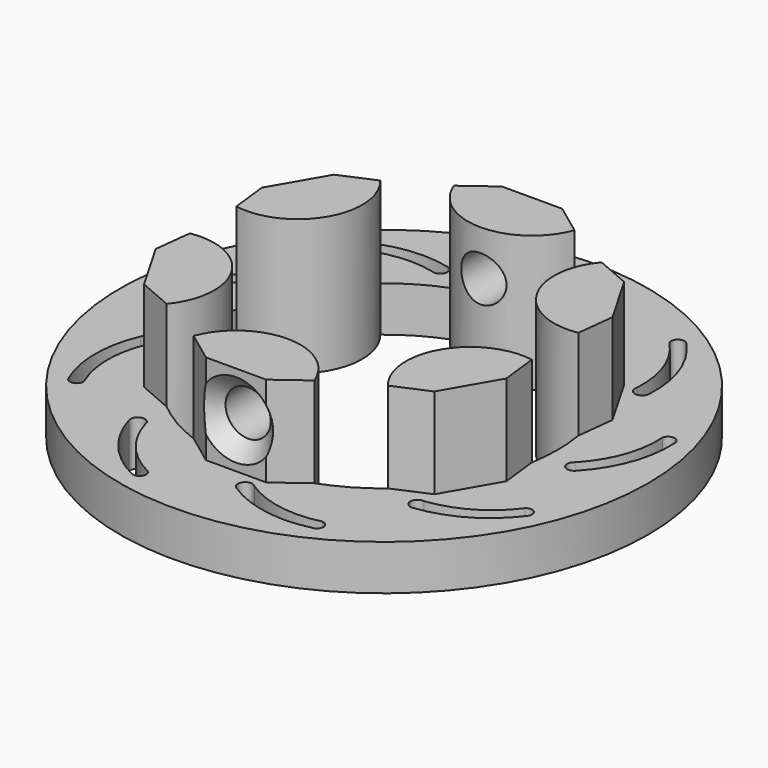
from build123d import *

# Parameters (mm, degrees)
F0_R          = 17.5
F0_R_2        = 11.5
F1_DEPTH      = 3
F3_DEPTH      = 3.001
F5_DEPTH      = 6
F5_DEPTH_BACK = 3
F6_R          = 1.5
F7_DEPTH      = 29.767666761


# Not quite as in the source:
# - a fillet or chamfer that OpenCascade refuses, or shapes differently, is made with other operations: its cross-section is extruded or revolved along the edge and cut away or added


with BuildPart() as f1:
    # F0 (on Top) → F1 (new body)
    with BuildSketch(Plane.XY):
        Circle(F0_R)
        Circle(F0_R_2, mode=Mode.SUBTRACT)
    extrude(amount=F1_DEPTH)

    # F2 (on Top) → F3 (cut, through all)
    with BuildSketch(Plane.XY):
        with BuildLine():
            ThreePointArc((10.3428791664, 8.0132342217), (10.722508829, 7.4074823165), (11.2842680034, 7.8496142891))
            ThreePointArc((11.2842680034, 7.8496142891), (10.8476709377, 10.9006538274), (9.2192751651, 13.5174813857))
            ThreePointArc((9.2192751651, 13.5174813857), (8.6315737781, 13.5584848298), (8.5342502168, 12.9774492654))
            ThreePointArc((8.5342502168, 12.9774492654), (9.9604845752, 10.6854945477), (10.3428791664, 8.0132342217))
        make_face()
        with BuildLine():
            ThreePointArc((2.7722974401, 12.7867681236), (3.4524804527, 12.5667564861), (3.5986159928, 13.2665410638))
            ThreePointArc((3.5986159928, 13.2665410638), (1.3029928249, 15.3231337636), (-1.6264950391, 16.2810273468))
            ThreePointArc((-1.6264950391, 16.2810273468), (-2.1030569267, 15.9346706376), (-1.8041286384, 15.427013193))
            ThreePointArc((-1.8041286384, 15.427013193), (0.761670361, 14.5880397916), (2.7722974401, 12.7867681236))
        make_face()
        with BuildLine():
            ThreePointArc((-6.0954730691, 11.5772311114), (-5.4330018975, 11.8459056319), (-5.770868435, 12.4759058335))
            ThreePointArc((-5.770868435, 12.4759058335), (-8.8513701119, 12.5757491141), (-11.711210138, 11.426499669))
            ThreePointArc((-11.711210138, 11.426499669), (-11.8536439226, 10.85484696), (-11.298335653, 10.6581061954))
            ThreePointArc((-11.298335653, 10.6581061954), (-8.7935378801, 11.6646790891), (-6.0954730691, 11.5772311114))
        make_face()
        with BuildLine():
            ThreePointArc((-12.1111039857, 4.9505789955), (-11.7763222787, 5.5822238799), (-12.440099386, 5.8476556095))
            ThreePointArc((-12.440099386, 5.8476556095), (-14.8640786012, 3.9440316902), (-16.3161198577, 1.2253858046))
            ThreePointArc((-16.3161198577, 1.2253858046), (-16.0577791885, 0.6959197515), (-15.5059258486, 0.9021528573))
            ThreePointArc((-15.5059258486, 0.9021528573), (-14.2341520178, 3.2832854023), (-12.1111039857, 4.9505789955))
        make_face()
        with BuildLine():
            ThreePointArc((-12.4598147474, -3.9925040519), (-12.6093705865, -3.293442465), (-13.288469578, -3.5167776637))
            ThreePointArc((-13.288469578, -3.5167776637), (-13.9217195173, -6.5331419945), (-13.2865357625, -9.5490996964))
            ThreePointArc((-13.2865357625, -9.5490996964), (-12.7483011098, -9.7886360429), (-12.4581210104, -9.275927829))
            ThreePointArc((-12.4581210104, -9.275927829), (-13.0144482314, -6.6343940139), (-12.4598147474, -3.9925040519))
        make_face()
        with BuildLine():
            ThreePointArc((-6.9784397134, -11.0674500817), (-7.5423542593, -10.6280704779), (-7.9190171696, -11.2356715834))
            ThreePointArc((-7.9190171696, -11.2356715834), (-6.4652331485, -13.9533859322), (-4.0400339207, -15.855455323))
            ThreePointArc((-4.0400339207, -15.855455323), (-3.4737512602, -15.6929802443), (-3.5810228949, -15.1136987937))
            ThreePointArc((-3.5810228949, -15.1136987937), (-5.705139478, -13.4477667379), (-6.9784397134, -11.0674500817))
        make_face()
        with BuildLine():
            ThreePointArc((1.7682248193, -12.9638132172), (1.0538134497, -12.9897061964), (1.1558313826, -13.6972698986))
            ThreePointArc((1.1558313826, -13.6972698986), (4.0164076635, -14.8446855176), (7.0968446926, -14.7428671903))
            ThreePointArc((7.0968446926, -14.7428671903), (7.4262054104, -14.2544045814), (6.9716756317, -13.8796021227))
            ThreePointArc((6.9716756317, -13.8796021227), (4.2736674427, -13.9687799499), (1.7682248193, -12.9638132172))
        make_face()
        with BuildLine():
            ThreePointArc((9.6875173073, -8.7942640717), (9.1568901338, -9.2733140211), (9.6898535852, -9.7497634001))
            ThreePointArc((9.6898535852, -9.7497634001), (12.6187266924, -8.7899917691), (14.9130308016, -6.7319276504))
            ThreePointArc((14.9130308016, -6.7319276504), (14.8513580365, -6.1460345947), (14.2622496488, -6.151085364))
            ThreePointArc((14.2622496488, -6.151085364), (12.2527778705, -7.9536457777), (9.6875173073, -8.7942640717))
        make_face()
        with BuildLine():
            ThreePointArc((13.0739127825, -0.5097810297), (12.9753561567, -1.2178351539), (13.6898856045, -1.2402342502))
            ThreePointArc((13.6898856045, -1.2402342502), (15.3166032603, 1.3776368181), (15.7512440587, 4.4289556541))
            ThreePointArc((15.7512440587, 4.4289556541), (15.3273951828, 4.8381332844), (14.8793585479, 4.4555925983))
            ThreePointArc((14.8793585479, 4.4555925983), (14.4986773582, 1.7830876488), (13.0739127825, -0.5097810297))
        make_face()
    extrude(amount=F3_DEPTH, mode=Mode.SUBTRACT)

    # F4 (on face) → F5 (join, two sides)
    with BuildSketch(Plane.XY.offset(3)) as f5_sk:
        with BuildLine():
            ThreePointArc((-4, 10.7819293264), (0, 8), (4, 10.7819293264))
            ThreePointArc((4, 10.7819293264), (0, 11.5), (-4, 10.7819293264))
        make_face()
        with BuildLine():
            ThreePointArc((7.3374246985, 8.8550662783), (6.9282032303, 4), (11.3374246985, 1.9268630481))
            ThreePointArc((11.3374246985, 1.9268630481), (9.9592921435, 5.75), (7.3374246985, 8.8550662783))
        make_face()
        with BuildLine():
            ThreePointArc((7.3374246985, -8.8550662783), (9.9592921435, -5.75), (11.3374246985, -1.9268630481))
            ThreePointArc((11.3374246985, -1.9268630481), (6.9282032303, -4), (7.3374246985, -8.8550662783))
        make_face()
        with BuildLine():
            ThreePointArc((-4, -10.7819293264), (0, -11.5), (4, -10.7819293264))
            ThreePointArc((4, -10.7819293264), (0, -8), (-4, -10.7819293264))
        make_face()
        with BuildLine():
            ThreePointArc((-11.3374246985, -1.9268630481), (-9.9592921435, -5.75), (-7.3374246985, -8.8550662783))
            ThreePointArc((-7.3374246985, -8.8550662783), (-6.9282032303, -4), (-11.3374246985, -1.9268630481))
        make_face()
        with BuildLine():
            ThreePointArc((-11.3374246985, 1.9268630481), (-6.9282032303, 4), (-7.3374246985, 8.8550662783))
            ThreePointArc((-7.3374246985, 8.8550662783), (-9.9592921435, 5.75), (-11.3374246985, 1.9268630481))
        make_face()
        with BuildLine():
            ThreePointArc((-4, 10.7819293264), (0, 11.5), (4, 10.7819293264))
            Line((4, 10.7819293264), (2, 12.266666761))
            Line((2, 12.266666761), (0, 12.266666761))
            Line((0, 12.266666761), (-2, 12.266666761))
            Line((-2, 12.266666761), (-4, 10.7819293264))
        make_face()
        with BuildLine():
            ThreePointArc((7.3374246985, 8.8550662783), (9.9592921435, 5.75), (11.3374246985, 1.9268630481))
            Line((11.3374246985, 1.9268630481), (11.6232450348, 4.4012825729))
            Line((11.6232450348, 4.4012825729), (10.6232450348, 6.1333333805))
            Line((10.6232450348, 6.1333333805), (9.6232450348, 7.8653841881))
            Line((9.6232450348, 7.8653841881), (7.3374246985, 8.8550662783))
        make_face()
        with BuildLine():
            Line((11.6232450348, -4.4012825729), (11.3374246985, -1.9268630481))
            ThreePointArc((11.3374246985, -1.9268630481), (9.9592921435, -5.75), (7.3374246985, -8.8550662783))
            Line((7.3374246985, -8.8550662783), (9.6232450348, -7.8653841881))
            Line((9.6232450348, -7.8653841881), (10.6232450348, -6.1333333805))
            Line((10.6232450348, -6.1333333805), (11.6232450348, -4.4012825729))
        make_face()
        with BuildLine():
            Line((2, -12.266666761), (4, -10.7819293264))
            ThreePointArc((4, -10.7819293264), (0, -11.5), (-4, -10.7819293264))
            Line((-4, -10.7819293264), (-2, -12.266666761))
            Line((-2, -12.266666761), (0, -12.266666761))
            Line((0, -12.266666761), (2, -12.266666761))
        make_face()
        with BuildLine():
            Line((-9.6232450348, -7.8653841881), (-7.3374246985, -8.8550662783))
            ThreePointArc((-7.3374246985, -8.8550662783), (-9.9592921435, -5.75), (-11.3374246985, -1.9268630481))
            Line((-11.3374246985, -1.9268630481), (-11.6232450348, -4.4012825729))
            Line((-11.6232450348, -4.4012825729), (-10.6232450348, -6.1333333805))
            Line((-10.6232450348, -6.1333333805), (-9.6232450348, -7.8653841881))
        make_face()
        with BuildLine():
            ThreePointArc((-11.3374246985, 1.9268630481), (-9.9592921435, 5.75), (-7.3374246985, 8.8550662783))
            Line((-7.3374246985, 8.8550662783), (-9.6232450348, 7.8653841881))
            Line((-9.6232450348, 7.8653841881), (-10.6232450348, 6.1333333805))
            Line((-10.6232450348, 6.1333333805), (-11.6232450348, 4.4012825729))
            Line((-11.6232450348, 4.4012825729), (-11.3374246985, 1.9268630481))
        make_face()
    extrude(amount=F5_DEPTH)
    extrude(f5_sk.sketch, amount=-F5_DEPTH_BACK)

    # F6 (on face) → F7 (cut, through all)
    with BuildSketch(Plane.XZ.offset(12.266666761)):
        with Locations((0, 6)):
            Circle(F6_R)
    extrude(amount=-F7_DEPTH, mode=Mode.SUBTRACT)

    # F8: chamfer of 1 on 2 edges, made by hand

    # F8_s1 → F8_t2 (revolve, cut)
    with BuildSketch(Plane.XY.offset(6)):
        Polygon((2.5, -12.266666761), (1.5, -11.266666761), (1.5, -12.266666761), align=None)
    revolve(axis=Axis((0, -12.266666761, 6), (0, -1, 0)), mode=Mode.SUBTRACT)

    # F8_s3 → F8_t4 (revolve, cut)
    with BuildSketch(Plane.XY.offset(6)):
        Polygon((2.5, 12.266666761), (1.5, 11.266666761), (1.5, 12.266666761), align=None)
    revolve(axis=Axis((0, 12.266666761, 6), (0, -1, 0)), mode=Mode.SUBTRACT)


solid = f1.part
